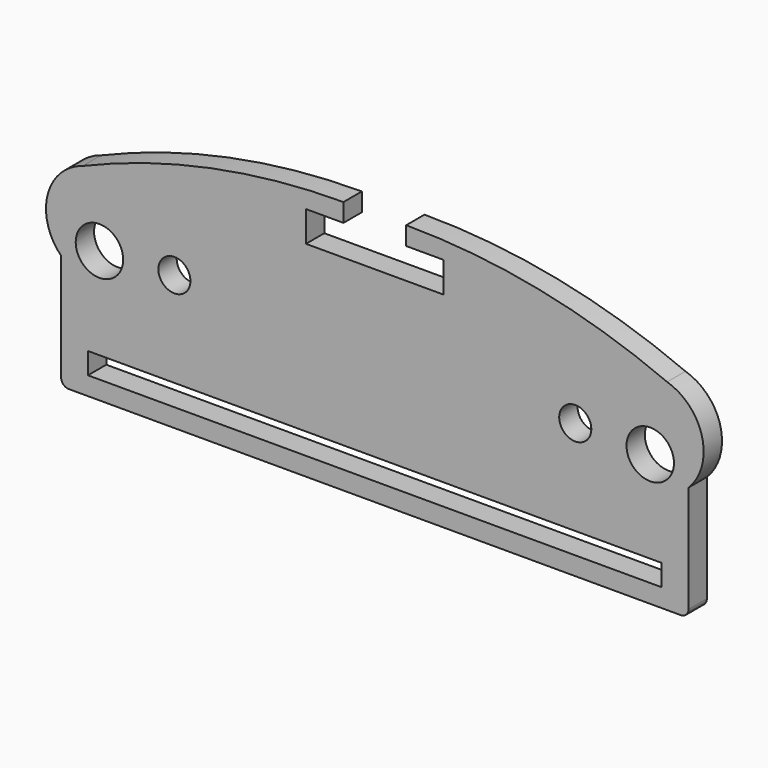
from build123d import *

# Parameters (mm, degrees)
F0_W      = 43
F0_H      = 16.6
F1_DEPTH  = 0.75
F2_W      = 37.5
F2_H      = 1.4
F3_DEPTH  = 75
F5_R      = 1.05
F5_R_2    = 1.55
F6_DEPTH  = 1.501
F7_W      = 4.1
F7_H      = 1.9489285067
F7_H_2    = 0.8016004696
F7_W_2    = 2
F7_H_3    = 15
F8_DEPTH  = 1.501
F10_DEPTH = 1.501
F11_R     = 0.5


# Not quite as in the source:
# - a feature of the source that left no trace in its solid (it failed there, or was rolled back) is left out
# - a pattern or mirror of a feature is missing from the dataset's text; its kind, count and spacing are read off the source's solid


with BuildPart() as f1:
    # F0 (on Front) → F1 (new body, symmetric)
    with BuildSketch(Plane.XZ):
        Rectangle(F0_W, F0_H)
    extrude(amount=F1_DEPTH, both=True)

    # F2 (on Front) → F3 (cut, symmetric)
    with BuildSketch(Plane.XZ):
        with Locations((0, -6.4)):
            Rectangle(F2_W, F2_H)
    extrude(amount=F3_DEPTH, both=True, mode=Mode.SUBTRACT)

    # F5 (on face) → F6 (cut, through all)
    with BuildSketch(Plane.XZ.offset(0.75)):
        with Locations((13.1, 0.5)):
            Circle(F5_R)
        with Locations((18, 0.3)):
            Circle(F5_R_2)
    f6 = extrude(amount=-F6_DEPTH, mode=Mode.SUBTRACT)

    # F6_copies: F6 across plane
    add(f6.mirror(Plane(origin=(0, 0, 0), x_dir=(0, 0, -1), z_dir=(-1, 0, 0))), mode=Mode.SUBTRACT)

    # F7 (on face) → F8 (cut, through all)
    with BuildSketch(Plane.XZ.offset(0.75)):
        Polygon((-2.05, 7.1), (-4.5, 7.1), (-4.5, 5.1), (4.5, 5.1), (4.5, 7.1), (2.05, 7.1), (2.05, 6.2983995304), (-2.05, 6.2983995304), align=None)
        with Locations((0, 8.0744642533)):
            Rectangle(F7_W, F7_H)
        with Locations((0, 6.6991997652)):
            Rectangle(F7_W, F7_H_2)
        with Locations((21.5, -8.3)):
            Rectangle(F7_W_2, F7_H_3)
    f8 = extrude(amount=-F8_DEPTH, mode=Mode.SUBTRACT)

    # F8_copies: F8 across plane
    add(f8.mirror(Plane(origin=(0, 0, 0), x_dir=(0, 0, -1), z_dir=(-1, 0, 0))), mode=Mode.SUBTRACT)

    # F9 (on face) → F10 (cut, through all)
    with BuildSketch(Plane.XZ.offset(0.75)):
        with BuildLine():
            ThreePointArc((2.05, 8.3), (10.75214793, 7.4237307967), (19.104892388, 4.8301066272))
            ThreePointArc((19.104892388, 4.8301066272), (21.392838702, 2.4091433089), (20.5, -0.8))
            Line((20.5, -0.8), (29.8848059028, -7.0995693095))
            Line((29.8848059028, -7.0995693095), (22.5688572973, 15.8109050244))
            Line((22.5688572973, 15.8109050244), (2.05, 8.3))
        make_face()
    f10 = extrude(amount=-F10_DEPTH, mode=Mode.SUBTRACT)

    # F10_copies: F10 across plane
    add(f10.mirror(Plane(origin=(0, 0, 0), x_dir=(0, 0, -1), z_dir=(-1, 0, 0))), mode=Mode.SUBTRACT)

    # F11
    f11_edges = [f1.edges().sort_by_distance(p)[0] for p in [
        (20.5, 0, -8.3),
        (-20.5, 0, -8.3),
    ]]
    fillet(f11_edges, radius=F11_R)


solid = f1.part
